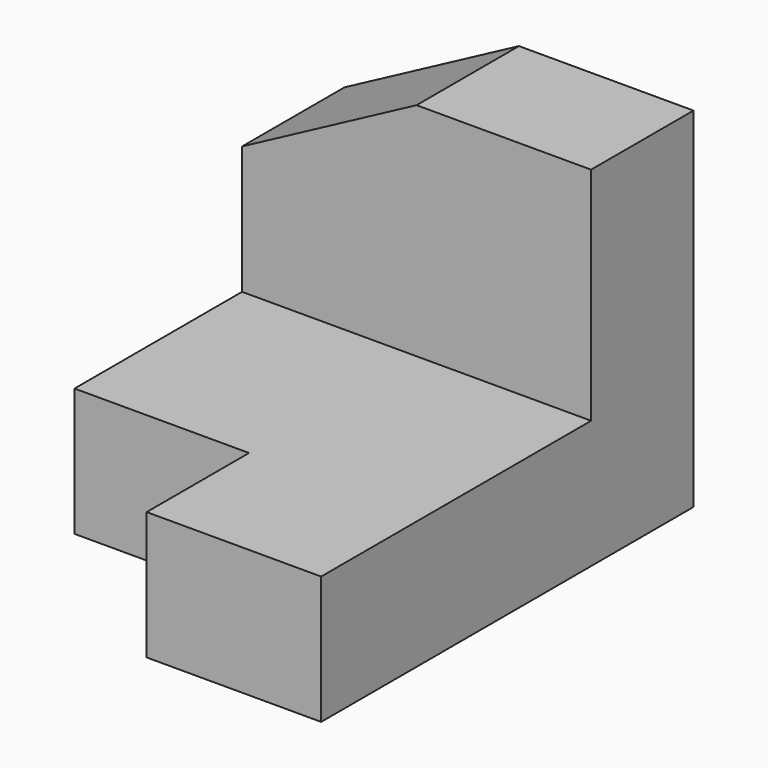
from build123d import *

# Parameters (mm, degrees)
F1_DEPTH = 30
F2_W     = 11
F2_H     = 15
F3_DEPTH = 11
F4_W     = 15
F4_H     = 8
F5_DEPTH = 11
F6_ANGLE = -90
F8_DEPTH = 11


with BuildPart() as f1:
    # F0 (on Front) → F1 (new body)
    with BuildSketch(Plane.XZ):
        Polygon((0, 30), (0, 0), (40, 0), (40, 11), (11, 11), (11, 30), align=None)
    extrude(amount=F1_DEPTH)

    # F2 (on face) → F3 (cut, through all)
    with BuildSketch(Plane.XY.offset(11)):
        with Locations((34.5, -22.5)):
            Rectangle(F2_W, F2_H)
    extrude(amount=-F3_DEPTH, mode=Mode.SUBTRACT)

    # F4 (on face) → F5 (cut, through all)
    with BuildSketch(Plane.YZ.offset(11)):
        with Locations((-22.5, 26)):
            Rectangle(F4_W, F4_H)
    extrude(amount=-F5_DEPTH, mode=Mode.SUBTRACT)


with BuildPart() as f1_1:
    # F6: moved
    add(f1.part.rotate(Axis((0, 0, 15), (0, 0, 1)), F6_ANGLE))

    # F7 (on face) → F8 (join, through all)
    with BuildSketch(Plane.XZ.offset(11)):
        Polygon((-15, 22), (-15, 30), (-30, 22), align=None)
    extrude(amount=-F8_DEPTH)


solid = f1_1.part
